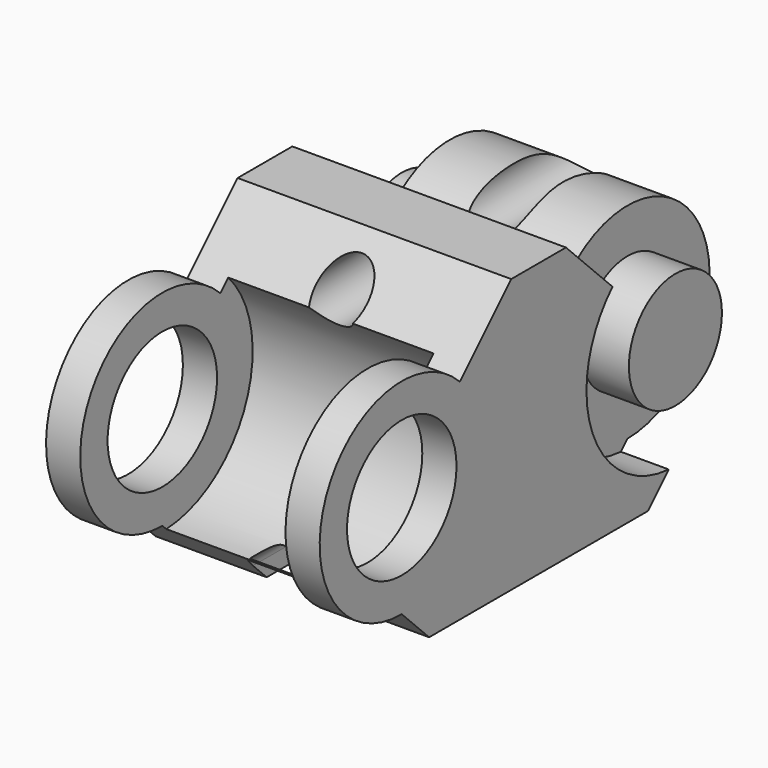
from build123d import *

# Parameters (mm, degrees)
F0_W          = 8
F0_H          = 10
F1_DEPTH      = 8
F2_SIZE       = 4
F4_DEPTH      = 4
F5_DEPTH      = 3
F6_R          = 3.3
F7_DEPTH      = 3
F9_DEPTH      = 1.4
F11_R         = 1.7
F12_DEPTH     = 4
F13_R         = 2
F14_DEPTH     = 12.5
F15_T1_DEPTH  = 13.1433659759
F15_T6_DEPTH  = 13.1433659759
F15_S7_R      = 3
F15_T8_DEPTH  = 8
F16_W         = 1.5
F16_H         = 1.0667801354
F16_H_2       = 8
F16_H_3       = 0.8089432385
F17_DEPTH     = 1
F18_T4_DEPTH  = 11.5268513298
F18_S7_R      = 3.3
F18_T8_DEPTH  = 7
F18_T12_DEPTH = 11.5268513298
F18_S14_R     = 3.3
F18_T15_DEPTH = 7
F19_R         = 0.75
F20_DEPTH     = 25


# Not quite as in the source:
# - a fillet or chamfer that OpenCascade refuses, or shapes differently, is made with other operations: its cross-section is extruded or revolved along the edge and cut away or added


with BuildPart() as f1:
    # F0 (on Top) → F1 (new body)
    with BuildSketch(Plane.XY):
        with Locations((0, 5)):
            Rectangle(F0_W, F0_H)
    extrude(amount=F1_DEPTH)

    # F2
    f2_edges = [f1.edges().sort_by_distance(p)[0] for p in [
        (0, 0, 8),
        (0, 10, 8),
    ]]
    chamfer(f2_edges, length=F2_SIZE)

    # F3 (on Right) → F4 (join, symmetric)
    with BuildSketch(Plane.YZ):
        with BuildLine():
            ThreePointArc((2.1213203436, 6.1213203436), (-2.7716385975, 5.1480502971), (0, 1))
            Line((0, 1), (0, 4))
            Line((0, 4), (2.1213203436, 6.1213203436))
        make_face()
    extrude(amount=F4_DEPTH, both=True)

    # F3 (on Right) → F5 (join, symmetric)
    with BuildSketch(Plane.YZ):
        with BuildLine():
            Line((10, 4), (10, 1))
            ThreePointArc((10, 1), (12.1213203436, 1.8786796564), (13, 4))
            ThreePointArc((13, 4), (11.1480502971, 6.7716385975), (7.8786796564, 6.1213203436))
            Line((7.8786796564, 6.1213203436), (10, 4))
        make_face()
    extrude(amount=F5_DEPTH, both=True)

    # F6 (on Right) → F7 (cut, symmetric)
    with BuildSketch(Plane.YZ):
        with Locations((0, 4.1532493821)):
            Circle(F6_R)
    extrude(amount=F7_DEPTH, both=True, mode=Mode.SUBTRACT)

    # F8 (on face) → F9 (cut)
    with BuildSketch(Plane(origin=(-4, 0, 0), x_dir=(0, -1, 0), z_dir=(-1, 0, 0))):
        with BuildLine():
            Line((-10, 4), (-7.7019029611, 6.2980970389))
            ThreePointArc((-7.7019029611, 6.2980970389), (-13.0026084807, 5.2437211552), (-10, 0.75))
            Line((-10, 0.75), (-10, 4))
        make_face()
        with BuildLine():
            ThreePointArc((-10, 0.75), (-7.7019029611, 1.7019029611), (-6.75, 4))
            ThreePointArc((-6.75, 4), (-6.9973915193, 5.2437211552), (-7.7019029611, 6.2980970389))
            Line((-7.7019029611, 6.2980970389), (-10, 4))
            Line((-10, 4), (-10, 0.75))
        make_face()
    extrude(amount=-F9_DEPTH, mode=Mode.SUBTRACT)

    # F10: F1 across plane


with BuildPart() as f1_1:
    add(f1.part)
    add(f1.part.mirror(Plane.YZ), mode=Mode.INTERSECT)

    # F11 (on Right) → F12 (join, symmetric)
    with BuildSketch(Plane.YZ):
        with Locations((10, 4)):
            Circle(F11_R)
    extrude(amount=F12_DEPTH, both=True)

    # F13 (on Right) → F14 (cut, symmetric)
    with BuildSketch(Plane.YZ):
        with Locations((0, 4)):
            Circle(F13_R)
    extrude(amount=F14_DEPTH, both=True, mode=Mode.SUBTRACT)

    # F15: chamfer of 1 on 2 edges, made by hand

    # F15_s2 → F15_t1 (cut)
    with BuildSketch(Plane.YZ.offset(-6.571682988)):
        Polygon((1, 0), (0, 1), (0, 0), align=None)
    extrude(amount=F15_T1_DEPTH, mode=Mode.SUBTRACT)


with BuildPart() as f15_tool4:
    # F15_s5 → F15_t6 (new body)
    with BuildSketch(Plane.YZ.offset(6.571682988)):
        Polygon((9, 0), (10, 1), (10, 0), align=None)
    extrude(amount=-F15_T6_DEPTH)

    # F15_s7 → F15_t8 (cut, symmetric)
    with BuildSketch(Plane.YZ):
        with Locations((10, 4)):
            Circle(F15_S7_R)
    extrude(amount=F15_T8_DEPTH, both=True, mode=Mode.SUBTRACT)


with BuildPart() as f1_2:
    add(f1_1.part)

    # F15_t3: cut F15_tool4
    add(f15_tool4.part, mode=Mode.SUBTRACT)

    # F16 (on face) → F17 (cut)
    with BuildSketch(Plane(origin=(0, 0, 0), x_dir=(1, 0, 0), z_dir=(0, 0, -1))):
        with Locations((0, -9.5333900677)):
            Rectangle(F16_W, F16_H)
        with Locations((0, -5)):
            Rectangle(F16_W, F16_H_2)
        with Locations((0, -0.5955283808)):
            Rectangle(F16_W, F16_H_3)
    extrude(amount=-F17_DEPTH, mode=Mode.SUBTRACT)

    # F18: fillet of radius 0.5 on 2 edges, made by hand


with BuildPart() as f18_tool2:
    # F18_s3 → F18_t4 (new body)
    with BuildSketch(Plane.XZ.offset(0.2768513298)):
        with BuildLine():
            ThreePointArc((-0.75, 0.5), (-0.6035533906, 0.8535533906), (-0.25, 1))
            Line((-0.25, 1), (-0.75, 1))
            Line((-0.75, 1), (-0.75, 0.5))
        make_face()
    extrude(amount=-F18_T4_DEPTH)

    split(bisect_by=Plane(origin=(0, 0.5, 0.5), x_dir=(1, 0, 0), z_dir=(0, 0.7071067812, 0.7071067812)), keep=Keep.TOP)

    split(bisect_by=Plane(origin=(0, 4.5, -4.5), x_dir=(1, 0, 0), z_dir=(0, -0.7071067812, 0.7071067812)), keep=Keep.TOP)

    # F18_s7 → F18_t8 (cut, symmetric)
    with BuildSketch(Plane.YZ.offset(-0.5)):
        with Locations((0, 4.1532493821)):
            Circle(F18_S7_R)
    extrude(amount=F18_T8_DEPTH, both=True, mode=Mode.SUBTRACT)


with BuildPart() as f1_3:
    add(f1_2.part)

    # F18_t1: union F18_tool2
    add(f18_tool2.part)


with BuildPart() as f18_tool10:
    # F18_s11 → F18_t12 (new body)
    with BuildSketch(Plane.XZ.offset(-11.25)):
        with BuildLine():
            ThreePointArc((0.75, 0.5), (0.6035533906, 0.8535533906), (0.25, 1))
            Line((0.25, 1), (0.75, 1))
            Line((0.75, 1), (0.75, 0.5))
        make_face()
    extrude(amount=F18_T12_DEPTH)

    split(bisect_by=Plane(origin=(0, 0.5, 0.5), x_dir=(1, 0, 0), z_dir=(0, 0.7071067812, 0.7071067812)), keep=Keep.TOP)

    # F18_s14 → F18_t15 (cut, symmetric)
    with BuildSketch(Plane.YZ.offset(0.5)):
        with Locations((0, 4.1532493821)):
            Circle(F18_S14_R)
    extrude(amount=F18_T15_DEPTH, both=True, mode=Mode.SUBTRACT)

    split(bisect_by=Plane(origin=(0, 4.5, -4.5), x_dir=(1, 0, 0), z_dir=(0, -0.7071067812, 0.7071067812)), keep=Keep.TOP)


with BuildPart() as f1_4:
    add(f1_3.part)

    # F18_t9: union F18_tool10
    add(f18_tool10.part)

    # F19 (on Front) → F20 (cut)
    with BuildSketch(Plane.XZ):
        with Locations((0, 6.8)):
            Circle(F19_R)
    extrude(amount=-F20_DEPTH, mode=Mode.SUBTRACT)


solid = f1_4.part
